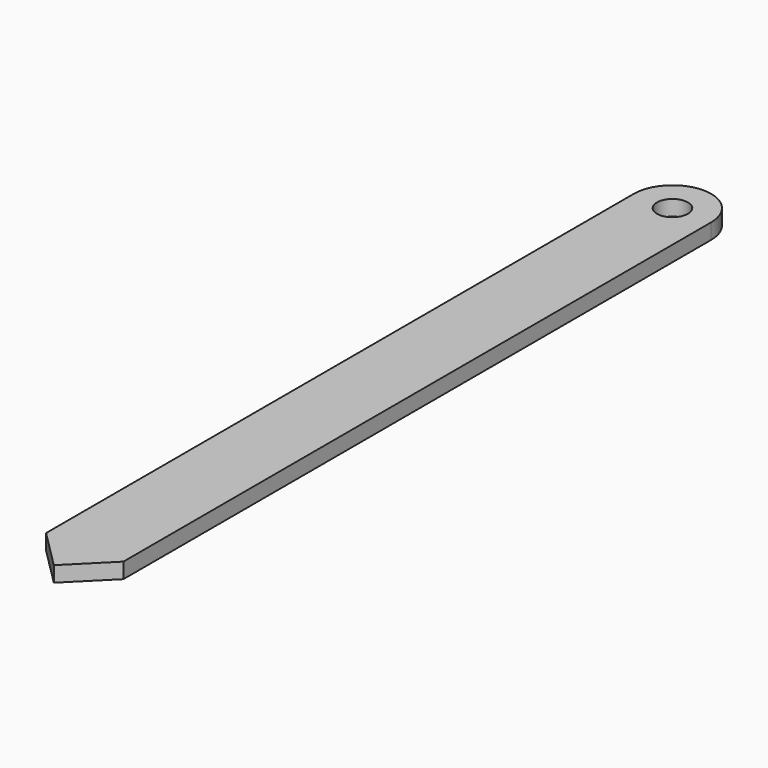
from build123d import *
from build123d import SkipClean  # not in build123d's __all__

# Parameters (mm, degrees)
F1_DEPTH = 10
F5_DEPTH = 10.001
F7_DEPTH = 10


with BuildPart() as f1:
    # F0 (on Top) → F1 (new body)
    with BuildSketch(Plane.XY):
        with BuildLine():
            Line((0, 240), (0, 0))
            Line((0, 0), (25, 0))
            Line((25, 0), (25, 250))
            ThreePointArc((25, 250), (17.6776695297, 267.6776695297), (0, 275))
            Line((0, 275), (0, 260))
            ThreePointArc((0, 260), (10, 250), (0, 240))
        make_face()
    extrude(amount=F1_DEPTH)

    # F2: F1 across face


with BuildPart() as f1_1:
    add(f1.part, clean=False)
    with SkipClean():  # cleaning this boolean's faces spoils the solid; the shape is the same uncleaned
        add(f1.part.mirror(Plane(origin=(0, 120, 5), x_dir=(0, -1, 0), z_dir=(-1, 0, 0))), clean=False)

    # F3: F1 across face


with BuildPart() as f1_2:
    add(f1_1.part, clean=False)
    add(f1_1.part.mirror(Plane(origin=(12.5, 0, 5), x_dir=(1, 0, 0), z_dir=(0, -1, 0))), clean=False)

    # F4 (on Top) → F5 (cut, through all)
    with BuildSketch(Plane.XY):
        Polygon((50, -200), (0, -250), (-50, -200), (-50, -344.7760872496), (50, -344.7760872496), align=None)
    extrude(amount=F5_DEPTH, mode=Mode.SUBTRACT)

    # F6 (on face) → F7 (join, through all)
    with BuildSketch(Plane.XY.offset(10)):
        Polygon((11.9149819948, -238.0850180052), (-11.0190114938, -238.9809885062), (0, -250), align=None)
    extrude(amount=-F7_DEPTH)


solid = f1_2.part
